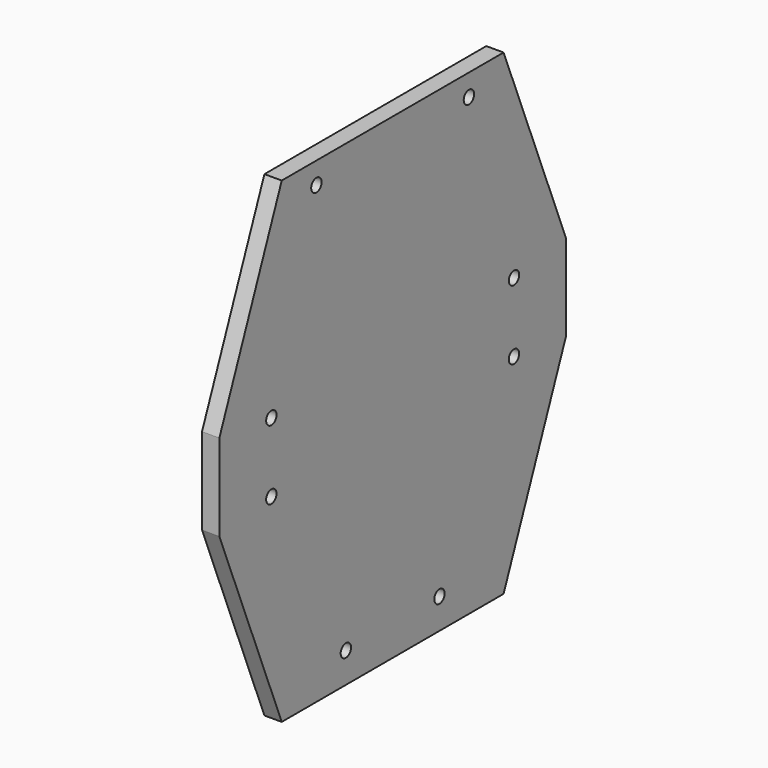
from build123d import *

# Parameters (mm, degrees)
F1_DEPTH = 4
F2_W     = 7.5
F2_H     = 6
F3_DEPTH = 28
F4_R     = 2.99999
F2_R     = 1.5
F5_DEPTH = 25


# Not quite as in the source:
# - a fillet or chamfer is up to 0.001 mm smaller than in the source, because OpenCascade refuses the exact size


with BuildPart() as f1:
    # F0 (on Right) → F1 (new body)
    with BuildSketch(Plane.YZ):
        Polygon((-50, 55), (0, 55), (0, 65), (-18, 110), (-50, 110), align=None)
        Polygon((-50, 0), (-18, 0), (0, 45), (0, 55), (-50, 55), align=None)
        Polygon((-100, 55), (-50, 55), (-50, 110), (-82, 110), (-100, 65), align=None)
        Polygon((-82, 0), (-50, 0), (-50, 55), (-100, 55), (-100, 45), align=None)
    extrude(amount=F1_DEPTH)

    # F2 (on face) → F3 (join)
    with BuildSketch(Plane(origin=(0, 0, 0), x_dir=(0, -1, 0), z_dir=(-1, 0, 0))):
        with Locations((53.75, 7)):
            Rectangle(F2_W, F2_H)
        Polygon((42.5, 4), (50, 4), (50, 10), (42.5, 10), (42.5, 7), align=None)
    extrude(amount=F3_DEPTH)

    # F4 (radius 3 in the source; OpenCascade refuses exactly that, so slightly less here)
    f4_edges = [f1.edges().sort_by_distance(p)[0] for p in [
        (-28, -50, 4),
        (-28, -50, 10),
    ]]
    fillet(f4_edges, radius=F4_R)

    # F2 (on face) → F5 (cut)
    with BuildSketch(Plane(origin=(0, 0, 0), x_dir=(0, -1, 0), z_dir=(-1, 0, 0))):
        with Locations((72, 105)):
            Circle(F2_R)
        with Locations((85, 63)):
            Circle(F2_R)
        with Locations((85, 47)):
            Circle(F2_R)
        with Locations((15, 63)):
            Circle(F2_R)
        with BuildLine():
            ThreePointArc((16.5, 47), (15, 48.5), (13.5, 47))
            ThreePointArc((13.5, 47), (15, 45.5), (16.5, 47))
        make_face()
        with BuildLine():
            ThreePointArc((29.5, 105), (29.0606601718, 106.0606601718), (28, 106.5))
            ThreePointArc((28, 106.5), (26.9393398282, 103.9393398282), (29.5, 105))
        make_face()
        with Locations((63.5, 7)):
            Circle(F2_R)
        with Locations((36.5, 7)):
            Circle(F2_R)
    extrude(amount=-F5_DEPTH, mode=Mode.SUBTRACT)


solid = f1.part
